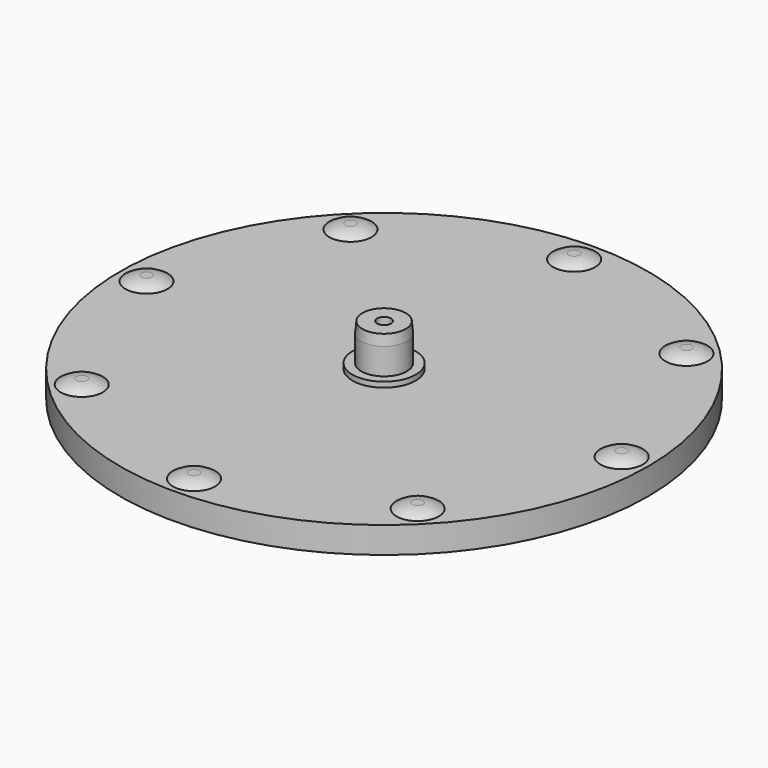
from build123d import *

# Parameters (mm, degrees)
F0_R      = 50
F1_DEPTH  = 5
F2_R      = 6
F3_DEPTH  = 1
F4_R      = 4.3
F5_DEPTH  = 7
F7_D      = 2.65
F7_DEPTH  = 5
F7_TIP    = 0.7961403202
F8_SIZE2  = 2
F8_SIZE   = 0.2
F9_R      = 4
F10_DEPTH = 1


# Not quite as in the source:
# - a fillet or chamfer that OpenCascade refuses, or shapes differently, is made with other operations: its cross-section is extruded or revolved along the edge and cut away or added


with BuildPart() as f1:
    # F0 (on Top) → F1 (new body)
    with BuildSketch(Plane.XY):
        Circle(F0_R)
    extrude(amount=F1_DEPTH)

    # F2 (on face) → F3 (join)
    with BuildSketch(Plane.XY.offset(5)):
        Circle(F2_R)
    extrude(amount=F3_DEPTH)

    # F4 (on face) → F5 (join)
    with BuildSketch(Plane.XY.offset(6)):
        Circle(F4_R)
    extrude(amount=F5_DEPTH)

    # F7
    with Locations(Plane.XY.offset(13)):
        with Locations((0, 0)):
            Hole(F7_D / 2, depth=F7_DEPTH)
            with Locations((0, 0, -(F7_DEPTH + F7_TIP / 2))):  # 118° drill point
                Cone(0, F7_D / 2, F7_TIP, mode=Mode.SUBTRACT)

    # F8
    f8_edges = [f1.edges().sort_by_distance(p)[0] for p in [
        (-4.3, 0, 13),
    ]]
    f8_side = f1.faces().sort_by_distance((-4.178378, 0, 13))[0]
    chamfer(f8_edges, length=F8_SIZE, length2=F8_SIZE2, reference=f8_side)

    # F9 (on face) → F10 (join)
    with BuildSketch(Plane.XY.offset(5)):
        with Locations((0, 45)):
            Circle(F9_R)
        with Locations((-31.8198051534, 31.8198051534)):
            Circle(F9_R)
        with Locations((-45, 0)):
            Circle(F9_R)
        with Locations((-31.8198051534, -31.8198051534)):
            Circle(F9_R)
        with Locations((0, -45)):
            Circle(F9_R)
        with Locations((31.8198051534, -31.8198051534)):
            Circle(F9_R)
        with Locations((45, 0)):
            Circle(F9_R)
        with Locations((31.8198051534, 31.8198051534)):
            Circle(F9_R)
    extrude(amount=F10_DEPTH)

    # F11: fillet of radius 5 on 8 edges, made by hand

    # F11_s1 → F11_t2 (revolve, cut)
    with BuildSketch(Plane.XZ.offset(45)):
        with BuildLine():
            ThreePointArc((4, 5), (2.5811388301, 5.7434164903), (1, 6))
            Line((1, 6), (4, 6))
            Line((4, 6), (4, 5))
        make_face()
    revolve(axis=Axis((0, -45, 6), (0, 0, 1)), mode=Mode.SUBTRACT)

    # F11_s3 → F11_t4 (revolve, cut)
    with BuildSketch(Plane.XZ.offset(31.8198051534)):
        with BuildLine():
            ThreePointArc((35.8198051534, 5), (34.4009439835, 5.7434164903), (32.8198051534, 6))
            Line((32.8198051534, 6), (35.8198051534, 6))
            Line((35.8198051534, 6), (35.8198051534, 5))
        make_face()
    revolve(axis=Axis((31.8198051534, -31.8198051534, 6), (0, 0, 1)), mode=Mode.SUBTRACT)

    # F11_s5 → F11_t6 (revolve, cut)
    with BuildSketch(Plane.XZ):
        with BuildLine():
            ThreePointArc((49, 5), (47.5811388301, 5.7434164903), (46, 6))
            Line((46, 6), (49, 6))
            Line((49, 6), (49, 5))
        make_face()
    revolve(axis=Axis((45, 0, 6), (0, 0, 1)), mode=Mode.SUBTRACT)

    # F11_s7 → F11_t8 (revolve, cut)
    with BuildSketch(Plane.XZ.offset(-31.8198051534)):
        with BuildLine():
            ThreePointArc((35.8198051534, 5), (34.4009439835, 5.7434164903), (32.8198051534, 6))
            Line((32.8198051534, 6), (35.8198051534, 6))
            Line((35.8198051534, 6), (35.8198051534, 5))
        make_face()
    revolve(axis=Axis((31.8198051534, 31.8198051534, 6), (0, 0, 1)), mode=Mode.SUBTRACT)

    # F11_s9 → F11_t10 (revolve, cut)
    with BuildSketch(Plane.XZ.offset(-45)):
        with BuildLine():
            ThreePointArc((4, 5), (2.5811388301, 5.7434164903), (1, 6))
            Line((1, 6), (4, 6))
            Line((4, 6), (4, 5))
        make_face()
    revolve(axis=Axis((0, 45, 6), (0, 0, 1)), mode=Mode.SUBTRACT)

    # F11_s11 → F11_t12 (revolve, cut)
    with BuildSketch(Plane.XZ.offset(-31.8198051534)):
        with BuildLine():
            ThreePointArc((-27.8198051534, 5), (-29.2386663233, 5.7434164903), (-30.8198051534, 6))
            Line((-30.8198051534, 6), (-27.8198051534, 6))
            Line((-27.8198051534, 6), (-27.8198051534, 5))
        make_face()
    revolve(axis=Axis((-31.8198051534, 31.8198051534, 6), (0, 0, 1)), mode=Mode.SUBTRACT)

    # F11_s13 → F11_t14 (revolve, cut)
    with BuildSketch(Plane.XZ):
        with BuildLine():
            ThreePointArc((-41, 5), (-42.4188611699, 5.7434164903), (-44, 6))
            Line((-44, 6), (-41, 6))
            Line((-41, 6), (-41, 5))
        make_face()
    revolve(axis=Axis((-45, 0, 6), (0, 0, 1)), mode=Mode.SUBTRACT)

    # F11_s15 → F11_t16 (revolve, cut)
    with BuildSketch(Plane.XZ.offset(31.8198051534)):
        with BuildLine():
            ThreePointArc((-27.8198051534, 5), (-29.2386663233, 5.7434164903), (-30.8198051534, 6))
            Line((-30.8198051534, 6), (-27.8198051534, 6))
            Line((-27.8198051534, 6), (-27.8198051534, 5))
        make_face()
    revolve(axis=Axis((-31.8198051534, -31.8198051534, 6), (0, 0, 1)), mode=Mode.SUBTRACT)


solid = f1.part
